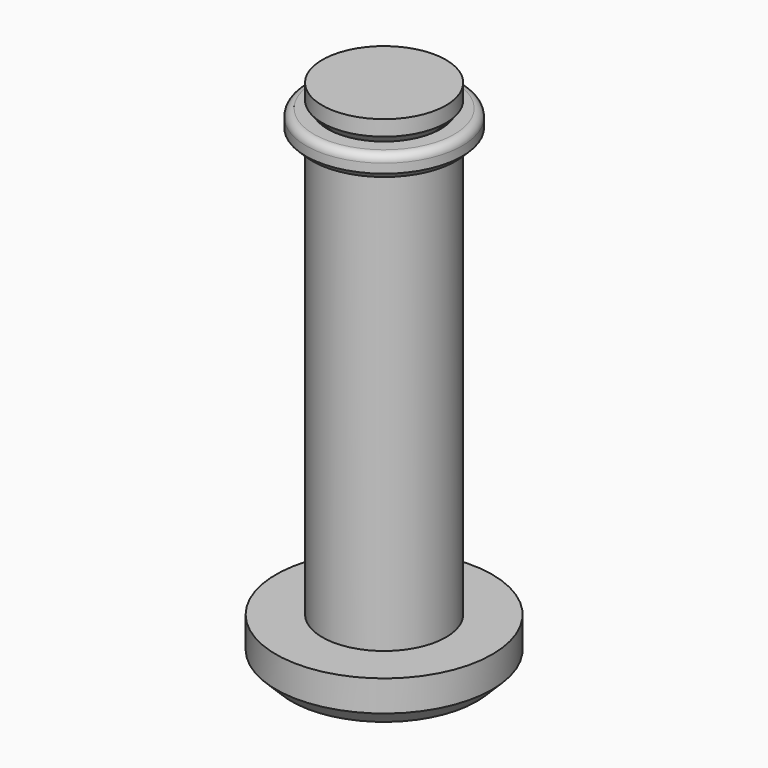
from build123d import *

# Parameters (mm, degrees)
F0_R         = 4
F1_DEPTH     = 30.3
F2_R         = 7
F3_DEPTH     = 3
F6_SIZE      = 1
F8_ANGLE     = 270
F9_R         = 2.6041880276
F10_T2_ANGLE = 298.457193056
F11_SIZE     = 0.4


# Not quite as in the source:
# - a fillet or chamfer that OpenCascade refuses, or shapes differently, is made with other operations: its cross-section is extruded or revolved along the edge and cut away or added


with BuildPart() as f1:
    # F0 (on Top) → F1 (new body)
    with BuildSketch(Plane.XY):
        Circle(F0_R)
    extrude(amount=F1_DEPTH)

    # F2 (on Top) → F3 (join)
    with BuildSketch(Plane.XY):
        Circle(F2_R)
    extrude(amount=-F3_DEPTH)

    # F4 (on Front) → F5 (revolve, cut)
    with BuildSketch(Plane.XZ):
        Polygon((-4, 29.3), (-4.1, 29.3), (-4.1, 27.3), (-3, 27.3), (-3, 28.3), align=None)
    revolve(axis=Axis((0, 0, 30.3), (0, 0, 1)), mode=Mode.SUBTRACT)

    # F6
    f6_edges = [f1.edges().sort_by_distance(p)[0] for p in [
        (-7, 0, -3),
    ]]
    chamfer(f6_edges, length=F6_SIZE)


with BuildPart() as f8:
    # F7 (on Front) → F8 (revolve)
    with BuildSketch(Plane.XZ):
        Polygon((-5.0517449093, 28.8404841072), (-5.0517449093, 27.3404841072), (-3.0517449093, 27.3404841072), (-3.0517449093, 28.2404841072), (-3.6517449093, 28.8404841072), align=None)
    revolve(axis=Axis((0, 0, 30.3), (0, 0, 1)), revolution_arc=F8_ANGLE)

    # F9
    f9_edges = [f8.edges().sort_by_distance(p)[0] for p in [
        (0, 3.051745, 27.790484),
        (-3.051745, 0, 27.790484),
    ]]
    fillet(f9_edges, radius=F9_R)

    # F10: fillet of radius 0.5 on 1 edges, made by hand

    # F10_s1 → F10_t2 (revolve, cut)
    with BuildSketch(Plane(origin=(0, 0, 0), x_dir=(0, 0, 1), z_dir=(0.2457912089, 0.9693227954, 0))):
        with BuildLine():
            ThreePointArc((28.8404841072, -4.5517449093), (28.6940374978, -4.9052982999), (28.3404841072, -5.0517449093))
            Line((28.3404841072, -5.0517449093), (28.8404841072, -5.0517449093))
            Line((28.8404841072, -5.0517449093), (28.8404841072, -4.5517449093))
        make_face()
    revolve(axis=Axis((0, 0, 28.8404841072), (0, 0, 1)), revolution_arc=F10_T2_ANGLE, mode=Mode.SUBTRACT)

    # F11
    f11_edges = [f8.edges().sort_by_distance(p)[0] for p in [
        (3.572123, -3.572123, 27.340484),
    ]]
    chamfer(f11_edges, length=F11_SIZE)


solid = Compound([f1.part, f8.part])
